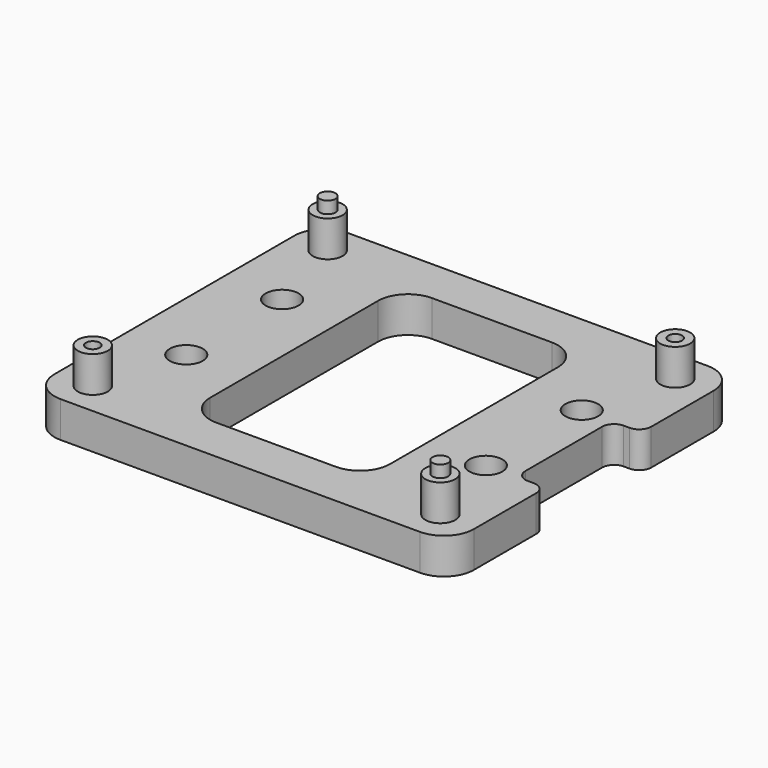
from build123d import *

# Parameters (mm, degrees)
F0_R     = 1.15
F0_R_2   = 2.75
F0_W     = 30
F0_H     = 45
F1_DEPTH = 6
F2_R     = 5
F4_R     = 2.5
F5_DEPTH = 6
F3_R     = 1.3
F6_DEPTH = 8
F7_R     = 1.15
F8_DEPTH = 25
F9_R     = 2


# Not quite as in the source:
# - a feature names something its author has since deleted; it is built from what else it names


with BuildPart() as f1:
    # F0 (on Top) → F1 (new body)
    with BuildSketch(Plane.XY):
        Polygon((35, 30), (-35, 30), (-35, -30), (35, -30), (35, -10), (30, -10), (30, 10), (35, 10), align=None)
        with Locations((-29, -24.5)):
            Circle(F0_R, mode=Mode.SUBTRACT)
        with Locations((-25, -10)):
            Circle(F0_R_2, mode=Mode.SUBTRACT)
        with Locations((25, -10)):
            Circle(F0_R_2, mode=Mode.SUBTRACT)
        with Locations((-25, 10)):
            Circle(F0_R_2, mode=Mode.SUBTRACT)
        Rectangle(F0_W, F0_H, mode=Mode.SUBTRACT)
        with Locations((25, 10)):
            Circle(F0_R_2, mode=Mode.SUBTRACT)
        with Locations((29, 24.5)):
            Circle(F0_R, mode=Mode.SUBTRACT)
    extrude(amount=F1_DEPTH)

    # F2
    f2_edges = [f1.edges().sort_by_distance(p)[0] for p in [
        (-35, -30, 3),
        (-35, 30, 3),
        (-15, 22.5, 3),
        (15, 22.5, 3),
        (15, -22.5, 3),
        (-15, -22.5, 3),
        (35, 30, 3),
        (35, -30, 3),
    ]]
    fillet(f2_edges, radius=F2_R)

    # F4 (on face) → F5 (join)
    with BuildSketch(Plane.XY.offset(6)):
        with Locations((-29, 24.5)):
            Circle(F4_R)
        with Locations((29, 24.5)):
            Circle(F4_R)
        with Locations((29, -24.5)):
            Circle(F4_R)
        with Locations((-29, -24.5)):
            Circle(F4_R)
    extrude(amount=F5_DEPTH)

    # F3 (on face) → F6 (join)
    with BuildSketch(Plane.XY.offset(6)):
        with Locations((-29, 24.5)):
            Circle(F3_R)
        with Locations((29, -24.5)):
            Circle(F3_R)
    extrude(amount=F6_DEPTH)

    # F7 (on face) → F8 (cut)
    with BuildSketch(Plane.XY.offset(12)):
        with Locations((-29, -24.5)):
            Circle(F7_R)
        with Locations((29, 24.5)):
            Circle(F7_R)
    extrude(amount=-F8_DEPTH, mode=Mode.SUBTRACT)

    # F9
    f9_edges = [f1.edges().sort_by_distance(p)[0] for p in [
        (35, 10, 3),
        (30, 10, 3),
        (30, -10, 3),
        (35, -10, 3),
    ]]
    fillet(f9_edges, radius=F9_R)


solid = f1.part
